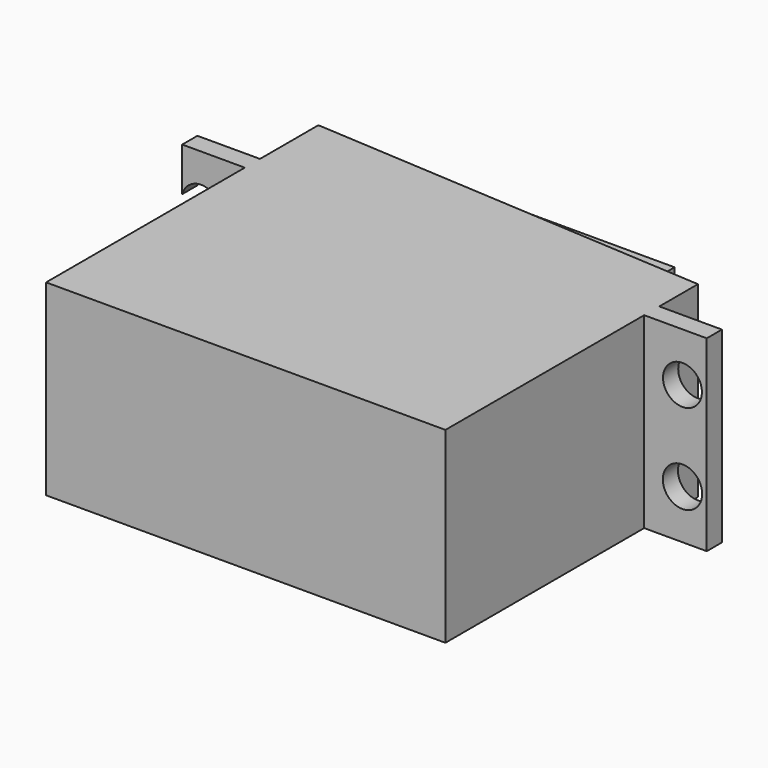
from build123d import *

# Parameters (mm, degrees)
F1_DEPTH = 9.885
F2_DEPTH = 8.905
F3_R     = 2.05
F3_R_2   = 2.075
F4_DEPTH = 25
F5_R     = 0.9
F6_DEPTH = 4.13


# Not quite as in the source:
# - a feature names something its author has since deleted; it is built from what else it names


with BuildPart() as f1:
    # F0 (on Top) → F1 (new body, symmetric)
    with BuildSketch(Plane.XY):
        Polygon((-4.56, 26.2), (-4.56, 0), (37.56, 0), (37.56, 26.2), (44.16, 26.2), (44.16, 28.2), (37.56, 28.2), (37.56, 33.2866495507), (33, 33.56957638), (0, 35.6170731707), (-4.56, 35.9), (-4.56, 28.2), (-11.16, 28.2), (-11.16, 26.2), align=None)
    extrude(amount=F1_DEPTH, both=True)

    # F0 (on Top) → F2 (join, symmetric)
    with BuildSketch(Plane.XY):
        Polygon((0, 35.9067581594), (0, 35.6170731707), (33, 33.56957638), (33, 35.9067581594), align=None)
    extrude(amount=F2_DEPTH, both=True)

    # F3 (on face) → F4 (cut)
    with BuildSketch(Plane(origin=(0, 28.2, 0), x_dir=(-1, 0, 0), z_dir=(0, 1, 0))):
        with Locations((9.16, -4.725)):
            Circle(F3_R)
        with Locations((9.16, 4.725)):
            Circle(F3_R_2)
        with Locations((-41.6, 4.725)):
            Circle(F3_R)
        with Locations((-41.6, -4.725)):
            Circle(F3_R_2)
    extrude(amount=-F4_DEPTH, mode=Mode.SUBTRACT)


with BuildPart() as f6:
    # F5 (on face) → F6 (new body)
    with BuildSketch(Plane(origin=(0, 35.9067581594, 0), x_dir=(-1, 0, 0), z_dir=(0, 1, 0))):
        with BuildLine():
            ThreePointArc((-28.6899656189, 1.033338959), (-28.6260791291, 1.1874039543), (-28.5534413217, 1.3375414089))
            Line((-28.5534413217, 1.3375414089), (-28.8418312249, 1.2937666255))
            Line((-28.8418312249, 1.2937666255), (-28.6899656189, 1.033338959))
        make_face()
        with BuildLine():
            ThreePointArc((-28.5390874953, 1.3648001419), (-28.4563953056, 1.5096431883), (-28.3655130563, 1.6494928329))
            Line((-28.3655130563, 1.6494928329), (-28.6571153541, 1.6422080659))
            Line((-28.6571153541, 1.6422080659), (-28.5390874953, 1.3648001419))
        make_face()
        with BuildLine():
            ThreePointArc((-28.347855989, 1.6747376112), (-28.2476622045, 1.8080744474), (-28.1399687808, 1.9354307696))
            Line((-28.1399687808, 1.9354307696), (-28.4301847307, 1.964750904))
            Line((-28.4301847307, 1.964750904), (-28.347855989, 1.6747376112))
        make_face()
        with BuildLine():
            ThreePointArc((-28.119286935, 1.9582634679), (-28.0031716716, 2.0779912923), (-27.8803654629, 2.1908458069))
            Line((-27.8803654629, 2.1908458069), (-28.1646181862, 2.2563084468))
            Line((-28.1646181862, 2.2563084468), (-28.119286935, 1.9582634679))
        make_face()
        with BuildLine():
            ThreePointArc((-27.8569850038, 2.2109063399), (-27.7267794685, 2.3151369733), (-27.5907972023, 2.4117098971))
            Line((-27.5907972023, 2.4117098971), (-27.8646038636, 2.5122826574))
            Line((-27.8646038636, 2.5122826574), (-27.8569850038, 2.2109063399))
        make_face()
        with BuildLine():
            ThreePointArc((-27.5650868536, 2.4286818982), (-27.4228444656, 2.5157715612), (-27.2758306633, 2.5945398815))
            Line((-27.2758306633, 2.5945398815), (-27.5348731681, 2.7286366698))
            Line((-27.5348731681, 2.7286366698), (-27.5650868536, 2.4286818982))
        make_face()
        with BuildLine():
            ThreePointArc((-27.2481958926, 2.6081556922), (-27.0961598992, 2.6767309287), (-26.9404330564, 2.736452422))
            Line((-26.9404330564, 2.736452422), (-27.1806261495, 2.9019584519))
            Line((-27.1806261495, 2.9019584519), (-27.2481958926, 2.6081556922))
        make_face()
        with BuildLine():
            ThreePointArc((-26.9113096805, 2.7464973129), (-26.7518777802, 2.7954766504), (-26.5898938022, 2.8352094732))
            Line((-26.5898938022, 2.8352094732), (-26.8074494952, 3.0295146156))
            Line((-26.8074494952, 3.0295146156), (-26.9113096805, 2.7464973129))
        make_face()
        with BuildLine():
            ThreePointArc((-26.5597411142, 2.8415250302), (-26.3954276433, 2.8701360355), (-26.2297411142, 2.8892535774))
            Line((-26.2297411142, 2.8892535774), (-26.4212284237, 3.1092935242))
            Line((-26.4212284237, 3.1092935242), (-26.5597411142, 2.8415250302))
        make_face()
        with BuildLine():
            ThreePointArc((-26.1990346399, 2.8917402004), (-26.03243092, 2.8995316607), (-25.8656548153, 2.8977324266))
            Line((-25.8656548153, 2.8977324266), (-26.0280538722, 3.1400370164))
            Line((-26.0280538722, 3.1400370164), (-26.1990346399, 2.8917402004))
        make_face()
        with BuildLine():
            ThreePointArc((-25.8348788143, 2.8963509002), (-25.6686122856, 2.8831999396), (-25.5033767641, 2.8605123045))
            Line((-25.5033767641, 2.8605123045), (-25.6341264382, 3.1212602492))
            Line((-25.6341264382, 3.1212602492), (-25.8348788143, 2.8963509002))
        make_face()
        with BuildLine():
            ThreePointArc((-25.4730165922, 2.8552844161), (-25.3097093771, 2.8213984331), (-25.1486203018, 2.7781801945))
            Line((-25.1486203018, 2.7781801945), (-25.2456585926, 3.0532593432))
            Line((-25.2456585926, 3.0532593432), (-25.4730165922, 2.8552844161))
        make_face()
        with BuildLine():
            ThreePointArc((-25.1191547571, 2.7691883911), (-24.961382308, 2.7151017878), (-24.8069801497, 2.6520345233))
            Line((-24.8069801497, 2.6520345233), (-24.8687767054, 2.9371067135))
            Line((-24.8687767054, 2.9371067135), (-25.1191547571, 2.7691883911))
        make_face()
        with BuildLine():
            ThreePointArc((-24.7788739214, 2.6394206109), (-24.6291244041, 2.5659863655), (-24.4838441771, 2.4840646834))
            Line((-24.4838441771, 2.4840646834), (-24.5094244291, 2.7746341564))
            Line((-24.5094244291, 2.7746341564), (-24.7788739214, 2.6394206109))
        make_face()
        with BuildLine():
            ThreePointArc((-24.4575405173, 2.468027591), (-24.3181755711, 2.3764038053), (-24.1843084314, 2.2769196595))
            Line((-24.1843084314, 2.2769196595), (-24.1732689638, 2.5684039611))
            Line((-24.1732689638, 2.5684039611), (-24.4575405173, 2.468027591))
        make_face()
        with BuildLine():
            ThreePointArc((-24.1602221644, 2.2577123016), (-24.0334396577, 2.1493439375), (-23.9130967701, 2.0338662524))
            Line((-23.9130967701, 2.0338662524), (-23.865611682, 2.3216685011))
            Line((-23.865611682, 2.3216685011), (-24.1602221644, 2.2577123016))
        make_face()
        with BuildLine():
            ThreePointArc((-23.8916077508, 2.0117915406), (-23.7794071196, 1.8883876318), (-23.6744863633, 1.7587375596))
            Line((-23.6744863633, 1.7587375596), (-23.5913045228, 2.0383189419))
            Line((-23.5913045228, 2.0383189419), (-23.8916077508, 2.0117915406))
        make_face()
        with BuildLine():
            ThreePointArc((-23.6559334863, 1.7341436251), (-23.5600842015, 1.5976503252), (-23.4722402395, 1.4558725248))
            Line((-23.4722402395, 1.4558725248), (-23.354673474, 1.7228238754))
            Line((-23.354673474, 1.7228238754), (-23.6559334863, 1.7341436251))
        make_face()
        with BuildLine():
            ThreePointArc((-23.4569160948, 1.4291472288), (-23.3789297569, 1.2817171185), (-23.3095479409, 1.1300475106))
            Line((-23.3095479409, 1.1300475106), (-23.1594503485, 1.3801588472))
            Line((-23.1594503485, 1.3801588472), (-23.4569160948, 1.4291472288))
        make_face()
        with BuildLine():
            ThreePointArc((-23.2976941995, 1.101612327), (-23.2388006996, 0.9455704672), (-23.1889752223, 0.7864009721))
            Line((-23.1889752223, 0.7864009721), (-23.0087139317, 1.0157278895))
            Line((-23.0087139317, 1.0157278895), (-23.2976941995, 1.101612327))
        make_face()
        with BuildLine():
            ThreePointArc((-23.1807788247, 0.7567043406), (-23.1419069485, 0.5945116047), (-23.1124235875, 0.4303524205))
            Line((-23.1124235875, 0.4303524205), (-22.9048414269, 0.6352782962))
            Line((-22.9048414269, 0.6352782962), (-23.1807788247, 0.7567043406))
        make_face()
        with BuildLine():
            ThreePointArc((-23.1080137957, 0.3998626748), (-23.0897765759, 0.2340769392), (-23.0811003014, 0.0675169542))
            Line((-23.0811003014, 0.0675169542), (-22.8494709655, 0.2448099847))
            Line((-22.8494709655, 0.2448099847), (-23.1080137957, 0.3998626748))
        make_face()
        with BuildLine():
            ThreePointArc((-23.0805466606, 0.0367149358), (-23.0803723456, 0.0183578357), (-23.0803142399, 0))
            ThreePointArc((-23.0803142399, 0), (-23.0841130057, -0.1483860211), (-23.0954993511, -0.2963832949))
            Line((-23.0954993511, -0.2963832949), (-22.8434757729, -0.1495191265))
            Line((-22.8434757729, -0.1495191265), (-23.0805466606, 0.0367149358))
        make_face()
        with BuildLine():
            Line((-22.8869503967, -0.5414902318), (-23.0988105925, -0.3270118197))
            ThreePointArc((-23.0988105925, -0.3270118197), (-23.1223755644, -0.4921245038), (-23.1553936549, -0.6556094023))
            Line((-23.1553936549, -0.6556094023), (-22.8869503967, -0.5414902318))
        make_face()
        with BuildLine():
            Line((-22.9792092163, -0.9249217126), (-23.1625175582, -0.6855814035))
            ThreePointArc((-23.1625175582, -0.6855814035), (-23.2065908198, -0.8464386506), (-23.2598386438, -1.0044961578))
            Line((-23.2598386438, -1.0044961578), (-22.9792092163, -0.9249217126))
        make_face()
        with BuildLine():
            Line((-23.1187972548, -1.2937666255), (-23.2706628609, -1.033338959))
            ThreePointArc((-23.2706628609, -1.033338959), (-23.3345493506, -1.1874039543), (-23.407187158, -1.3375414089))
            Line((-23.407187158, -1.3375414089), (-23.1187972548, -1.2937666255))
        make_face()
        with BuildLine():
            Line((-23.3035131256, -1.6422080659), (-23.4215409844, -1.3648001419))
            ThreePointArc((-23.4215409844, -1.3648001419), (-23.5042331741, -1.5096431883), (-23.5951154234, -1.6494928329))
            Line((-23.5951154234, -1.6494928329), (-23.3035131256, -1.6422080659))
        make_face()
        with BuildLine():
            Line((-23.530443749, -1.964750904), (-23.6127724907, -1.6747376112))
            ThreePointArc((-23.6127724907, -1.6747376112), (-23.7129662752, -1.8080744474), (-23.820659699, -1.9354307696))
            Line((-23.820659699, -1.9354307696), (-23.530443749, -1.964750904))
        make_face()
        with BuildLine():
            Line((-23.7960102935, -2.2563084468), (-23.8413415448, -1.9582634679))
            ThreePointArc((-23.8413415448, -1.9582634679), (-23.9574568082, -2.0779912923), (-24.0802630168, -2.1908458069))
            Line((-24.0802630168, -2.1908458069), (-23.7960102935, -2.2563084468))
        make_face()
        with BuildLine():
            Line((-24.0960246161, -2.5122826574), (-24.1036434759, -2.2109063399))
            ThreePointArc((-24.1036434759, -2.2109063399), (-24.2338490112, -2.3151369733), (-24.3698312774, -2.4117098971))
            Line((-24.3698312774, -2.4117098971), (-24.0960246161, -2.5122826574))
        make_face()
        with BuildLine():
            Line((-24.4257553117, -2.7286366698), (-24.3955416261, -2.4286818982))
            ThreePointArc((-24.3955416261, -2.4286818982), (-24.5377840142, -2.5157715612), (-24.6847978164, -2.5945398815))
            Line((-24.6847978164, -2.5945398815), (-24.4257553117, -2.7286366698))
        make_face()
        with BuildLine():
            Line((-24.7800023302, -2.9019584519), (-24.7124325872, -2.6081556922))
            ThreePointArc((-24.7124325872, -2.6081556922), (-24.8644685805, -2.6767309287), (-25.0201954233, -2.736452422))
            Line((-25.0201954233, -2.736452422), (-24.7800023302, -2.9019584519))
        make_face()
        with BuildLine():
            Line((-25.1531789846, -3.0295146156), (-25.0493187992, -2.7464973129))
            ThreePointArc((-25.0493187992, -2.7464973129), (-25.2087506995, -2.7954766504), (-25.3707346775, -2.8352094732))
            Line((-25.3707346775, -2.8352094732), (-25.1531789846, -3.0295146156))
        make_face()
        with BuildLine():
            Line((-25.539400056, -3.1092935242), (-25.4008873656, -2.8415250302))
            ThreePointArc((-25.4008873656, -2.8415250302), (-25.5652008364, -2.8701360355), (-25.7308873656, -2.8892535774))
            Line((-25.7308873656, -2.8892535774), (-25.539400056, -3.1092935242))
        make_face()
        with BuildLine():
            Line((-25.9325746075, -3.1400370164), (-25.7615938398, -2.8917402004))
            ThreePointArc((-25.7615938398, -2.8917402004), (-25.9281975597, -2.8995316607), (-26.0949736644, -2.8977324266))
            Line((-26.0949736644, -2.8977324266), (-25.9325746075, -3.1400370164))
        make_face()
        with BuildLine():
            Line((-26.7149698872, -3.0532593432), (-26.4876118875, -2.8552844161))
            ThreePointArc((-26.4876118875, -2.8552844161), (-26.6509191026, -2.8213984331), (-26.8120081779, -2.7781801945))
            Line((-26.8120081779, -2.7781801945), (-26.7149698872, -3.0532593432))
        make_face()
        with BuildLine():
            ThreePointArc((-28.7981109215, 0.6855814035), (-28.7540376599, 0.8464386506), (-28.7007898359, 1.0044961578))
            Line((-28.7007898359, 1.0044961578), (-28.9814192634, 0.9249217126))
            Line((-28.9814192634, 0.9249217126), (-28.7981109215, 0.6855814035))
        make_face()
        with BuildLine():
            ThreePointArc((-28.8618178872, 0.3270118197), (-28.8382529153, 0.4921245038), (-28.8052348249, 0.6556094023))
            Line((-28.8052348249, 0.6556094023), (-29.073678083, 0.5414902318))
            Line((-29.073678083, 0.5414902318), (-28.8618178872, 0.3270118197))
        make_face()
        with BuildLine():
            Line((-29.1111575142, -0.2448099847), (-28.852614684, -0.3998626748))
            ThreePointArc((-28.852614684, -0.3998626748), (-28.8708519038, -0.2340769392), (-28.8795281783, -0.0675169542))
            Line((-28.8795281783, -0.0675169542), (-29.1111575142, -0.2448099847))
        make_face()
        with BuildLine():
            Line((-29.0557870528, -0.6352782962), (-28.779849655, -0.7567043406))
            ThreePointArc((-28.779849655, -0.7567043406), (-28.8187215313, -0.5945116047), (-28.8482048923, -0.4303524205))
            Line((-28.8482048923, -0.4303524205), (-29.0557870528, -0.6352782962))
        make_face()
        with BuildLine():
            Line((-28.951914548, -1.0157278895), (-28.6629342803, -1.101612327))
            ThreePointArc((-28.6629342803, -1.101612327), (-28.7218277802, -0.9455704672), (-28.7716532574, -0.7864009721))
            Line((-28.7716532574, -0.7864009721), (-28.951914548, -1.0157278895))
        make_face()
        with BuildLine():
            Line((-28.8011781312, -1.3801588472), (-28.5037123849, -1.4291472288))
            ThreePointArc((-28.5037123849, -1.4291472288), (-28.5816987228, -1.2817171185), (-28.6510805388, -1.1300475106))
            Line((-28.6510805388, -1.1300475106), (-28.8011781312, -1.3801588472))
        make_face()
        with BuildLine():
            ThreePointArc((-23.0954993511, -0.2963832949), (-23.0841130057, -0.1483860211), (-23.0803142399, 0))
            ThreePointArc((-23.0803142399, 0), (-23.0803723456, 0.0183578357), (-23.0805466606, 0.0367149358))
            ThreePointArc((-23.0805466606, 0.0367149358), (-23.0807825791, 0.0521166802), (-23.0811003014, 0.0675169542))
            ThreePointArc((-23.0811003014, 0.0675169542), (-23.0897765759, 0.2340769392), (-23.1080137957, 0.3998626748))
            ThreePointArc((-23.1080137957, 0.3998626748), (-23.1101782044, 0.4151134034), (-23.1124235875, 0.4303524205))
            ThreePointArc((-23.1124235875, 0.4303524205), (-23.1419069485, 0.5945116047), (-23.1807788247, 0.7567043406))
            ThreePointArc((-23.1807788247, 0.7567043406), (-23.1848375894, 0.7715635404), (-23.1889752223, 0.7864009721))
            ThreePointArc((-23.1889752223, 0.7864009721), (-23.2388006996, 0.9455704672), (-23.2976941995, 1.101612327))
            ThreePointArc((-23.2976941995, 1.101612327), (-23.3035833112, 1.1158456593), (-23.3095479409, 1.1300475106))
            ThreePointArc((-23.3095479409, 1.1300475106), (-23.3789297569, 1.2817171185), (-23.4569160948, 1.4291472288))
            ThreePointArc((-23.4569160948, 1.4291472288), (-23.4645426787, 1.4425302257), (-23.4722402395, 1.4558725248))
            ThreePointArc((-23.4722402395, 1.4558725248), (-23.5600842015, 1.5976503252), (-23.6559334863, 1.7341436251))
            ThreePointArc((-23.6559334863, 1.7341436251), (-23.6651772666, 1.7464652287), (-23.6744863633, 1.7587375596))
            ThreePointArc((-23.6744863633, 1.7587375596), (-23.7794071196, 1.8883876318), (-23.8916077508, 2.0117915406))
            ThreePointArc((-23.8916077508, 2.0117915406), (-23.9023229475, 2.0228574317), (-23.9130967701, 2.0338662524))
            ThreePointArc((-23.9130967701, 2.0338662524), (-24.0334396577, 2.1493439375), (-24.1602221644, 2.2577123016))
            ThreePointArc((-24.1602221644, 2.2577123016), (-24.1722397925, 2.2673479646), (-24.1843084314, 2.2769196595))
            ThreePointArc((-24.1843084314, 2.2769196595), (-24.3181755711, 2.3764038053), (-24.4575405173, 2.468027591))
            ThreePointArc((-24.4575405173, 2.468027591), (-24.4706710516, 2.4760810657), (-24.4838441771, 2.4840646834))
            ThreePointArc((-24.4838441771, 2.4840646834), (-24.6291244041, 2.5659863655), (-24.7788739214, 2.6394206109))
            ThreePointArc((-24.7788739214, 2.6394206109), (-24.7929102856, 2.6457648893), (-24.8069801497, 2.6520345233))
            ThreePointArc((-24.8069801497, 2.6520345233), (-24.961382308, 2.7151017878), (-25.1191547571, 2.7691883911))
            ThreePointArc((-25.1191547571, 2.7691883911), (-25.1338755892, 2.77372342), (-25.1486203018, 2.7781801945))
            ThreePointArc((-25.1486203018, 2.7781801945), (-25.3097093771, 2.8213984331), (-25.4730165922, 2.8552844161))
            ThreePointArc((-25.4730165922, 2.8552844161), (-25.4881897361, 2.8579386755), (-25.5033767641, 2.8605123045))
            ThreePointArc((-25.5033767641, 2.8605123045), (-25.6686122856, 2.8831999396), (-25.8348788143, 2.8963509002))
            ThreePointArc((-25.8348788143, 2.8963509002), (-25.8502649803, 2.8970825308), (-25.8656548153, 2.8977324266))
            ThreePointArc((-25.8656548153, 2.8977324266), (-26.03243092, 2.8995316607), (-26.1990346399, 2.8917402004))
            ThreePointArc((-26.1990346399, 2.8917402004), (-26.214391179, 2.8905376639), (-26.2297411142, 2.8892535774))
            ThreePointArc((-26.2297411142, 2.8892535774), (-26.3954276433, 2.8701360355), (-26.5597411142, 2.8415250302))
            ThreePointArc((-26.5597411142, 2.8415250302), (-26.5748258446, 2.8384072914), (-26.5898938022, 2.8352094732))
            ThreePointArc((-26.5898938022, 2.8352094732), (-26.7518777802, 2.7954766504), (-26.9113096805, 2.7464973129))
            ThreePointArc((-26.9113096805, 2.7464973129), (-26.925884707, 2.7415135403), (-26.9404330564, 2.736452422))
            ThreePointArc((-26.9404330564, 2.736452422), (-27.0961598992, 2.6767309287), (-27.2481958926, 2.6081556922))
            ThreePointArc((-27.2481958926, 2.6081556922), (-27.2620313583, 2.601384483), (-27.2758306633, 2.5945398815))
            ThreePointArc((-27.2758306633, 2.5945398815), (-27.4228444656, 2.5157715612), (-27.5650868536, 2.4286818982))
            ThreePointArc((-27.5650868536, 2.4286818982), (-27.577964565, 2.4202300384), (-27.5907972023, 2.4117098971))
            ThreePointArc((-27.5907972023, 2.4117098971), (-27.7267794685, 2.3151369733), (-27.8569850038, 2.2109063399))
            ThreePointArc((-27.8569850038, 2.2109063399), (-27.8687018717, 2.2009071203), (-27.8803654629, 2.1908458069))
            ThreePointArc((-27.8803654629, 2.1908458069), (-28.0031716716, 2.0779912923), (-28.119286935, 1.9582634679))
            ThreePointArc((-28.119286935, 1.9582634679), (-28.1296581773, 1.9468745821), (-28.1399687808, 1.9354307696))
            ThreePointArc((-28.1399687808, 1.9354307696), (-28.2476622045, 1.8080744474), (-28.347855989, 1.6747376112))
            ThreePointArc((-28.347855989, 1.6747376112), (-28.3567180451, 1.6621386688), (-28.3655130563, 1.6494928329))
            ThreePointArc((-28.3655130563, 1.6494928329), (-28.4563953056, 1.5096431883), (-28.5390874953, 1.3648001419))
            ThreePointArc((-28.5390874953, 1.3648001419), (-28.5463006053, 1.3511898358), (-28.5534413217, 1.3375414089))
            ThreePointArc((-28.5534413217, 1.3375414089), (-28.6260791291, 1.1874039543), (-28.6899656189, 1.033338959))
            ThreePointArc((-28.6899656189, 1.033338959), (-28.6954160277, 1.0189319319), (-28.7007898359, 1.0044961578))
            ThreePointArc((-28.7007898359, 1.0044961578), (-28.7540376599, 0.8464386506), (-28.7981109215, 0.6855814035))
            ThreePointArc((-28.7981109215, 0.6855814035), (-28.8017126729, 0.6706048627), (-28.8052348249, 0.6556094023))
            ThreePointArc((-28.8052348249, 0.6556094023), (-28.8382529153, 0.4921245038), (-28.8618178872, 0.3270118197))
            ThreePointArc((-28.8618178872, 0.3270118197), (-28.8635141795, 0.3117019543), (-28.8651291286, 0.2963832949))
            ThreePointArc((-28.8651291286, 0.2963832949), (-28.8773967706, 0.1300492596), (-28.8800818191, -0.0367149358))
            ThreePointArc((-28.8800818191, -0.0367149358), (-28.8798459006, -0.0521166802), (-28.8795281783, -0.0675169542))
            ThreePointArc((-28.8795281783, -0.0675169542), (-28.8708519038, -0.2340769392), (-28.852614684, -0.3998626748))
            ThreePointArc((-28.852614684, -0.3998626748), (-28.8504502754, -0.4151134034), (-28.8482048923, -0.4303524205))
            ThreePointArc((-28.8482048923, -0.4303524205), (-28.8187215313, -0.5945116047), (-28.779849655, -0.7567043406))
            ThreePointArc((-28.779849655, -0.7567043406), (-28.7757908903, -0.7715635403), (-28.7716532574, -0.7864009721))
            ThreePointArc((-28.7716532574, -0.7864009721), (-28.7218277802, -0.9455704672), (-28.6629342803, -1.101612327))
            ThreePointArc((-28.6629342803, -1.101612327), (-28.6570451685, -1.1158456593), (-28.6510805388, -1.1300475106))
            ThreePointArc((-28.6510805388, -1.1300475106), (-28.5816987228, -1.2817171185), (-28.5037123849, -1.4291472288))
            ThreePointArc((-28.5037123849, -1.4291472288), (-28.496085801, -1.4425302257), (-28.4883882403, -1.4558725248))
            ThreePointArc((-28.4883882403, -1.4558725248), (-28.4005442782, -1.5976503252), (-28.3046949934, -1.7341436251))
            ThreePointArc((-28.3046949934, -1.7341436251), (-28.2954512131, -1.7464652287), (-28.2861421165, -1.7587375596))
            ThreePointArc((-28.2861421165, -1.7587375596), (-28.1812213601, -1.8883876318), (-28.0690207289, -2.0117915406))
            ThreePointArc((-28.0690207289, -2.0117915406), (-28.0583055322, -2.0228574317), (-28.0475317096, -2.0338662524))
            ThreePointArc((-28.0475317096, -2.0338662524), (-27.927188822, -2.1493439375), (-27.8004063153, -2.2577123016))
            ThreePointArc((-27.8004063153, -2.2577123016), (-27.7883886872, -2.2673479646), (-27.7763200483, -2.2769196595))
            ThreePointArc((-27.7763200483, -2.2769196595), (-27.6424529087, -2.3764038053), (-27.5030879625, -2.468027591))
            ThreePointArc((-27.5030879625, -2.468027591), (-27.4899574281, -2.4760810657), (-27.4767843026, -2.4840646834))
            ThreePointArc((-27.4767843026, -2.4840646834), (-27.3315040756, -2.5659863655), (-27.1817545583, -2.6394206109))
            ThreePointArc((-27.1817545583, -2.6394206109), (-27.1677181942, -2.6457648893), (-27.15364833, -2.6520345233))
            ThreePointArc((-27.15364833, -2.6520345233), (-26.9992461717, -2.7151017878), (-26.8414737227, -2.7691883911))
            ThreePointArc((-26.8414737227, -2.7691883911), (-26.8267528905, -2.77372342), (-26.8120081779, -2.7781801945))
            ThreePointArc((-26.8120081779, -2.7781801945), (-26.6509191026, -2.8213984331), (-26.4876118875, -2.8552844161))
            ThreePointArc((-26.4876118875, -2.8552844161), (-26.4724387437, -2.8579386755), (-26.4572517156, -2.8605123045))
            ThreePointArc((-26.4572517156, -2.8605123045), (-26.2920161942, -2.8831999396), (-26.1257496654, -2.8963509002))
            ThreePointArc((-26.1257496654, -2.8963509002), (-26.1103634994, -2.8970825308), (-26.0949736644, -2.8977324266))
            ThreePointArc((-26.0949736644, -2.8977324266), (-25.9281975597, -2.8995316607), (-25.7615938398, -2.8917402004))
            ThreePointArc((-25.7615938398, -2.8917402004), (-25.7462373007, -2.8905376639), (-25.7308873656, -2.8892535774))
            ThreePointArc((-25.7308873656, -2.8892535774), (-25.5652008364, -2.8701360355), (-25.4008873656, -2.8415250302))
            ThreePointArc((-25.4008873656, -2.8415250302), (-25.3858026351, -2.8384072914), (-25.3707346775, -2.8352094732))
            ThreePointArc((-25.3707346775, -2.8352094732), (-25.2087506995, -2.7954766504), (-25.0493187992, -2.7464973129))
            ThreePointArc((-25.0493187992, -2.7464973129), (-25.0347437727, -2.7415135403), (-25.0201954233, -2.736452422))
            ThreePointArc((-25.0201954233, -2.736452422), (-24.8644685805, -2.6767309287), (-24.7124325872, -2.6081556922))
            ThreePointArc((-24.7124325872, -2.6081556922), (-24.6985971214, -2.601384483), (-24.6847978164, -2.5945398815))
            ThreePointArc((-24.6847978164, -2.5945398815), (-24.5377840142, -2.5157715612), (-24.3955416261, -2.4286818982))
            ThreePointArc((-24.3955416261, -2.4286818982), (-24.3826639147, -2.4202300384), (-24.3698312774, -2.4117098971))
            ThreePointArc((-24.3698312774, -2.4117098971), (-24.2338490112, -2.3151369733), (-24.1036434759, -2.2109063399))
            ThreePointArc((-24.1036434759, -2.2109063399), (-24.091926608, -2.2009071203), (-24.0802630168, -2.1908458069))
            ThreePointArc((-24.0802630168, -2.1908458069), (-23.9574568082, -2.0779912923), (-23.8413415448, -1.9582634679))
            ThreePointArc((-23.8413415448, -1.9582634679), (-23.8309703024, -1.9468745821), (-23.820659699, -1.9354307696))
            ThreePointArc((-23.820659699, -1.9354307696), (-23.7129662752, -1.8080744474), (-23.6127724907, -1.6747376112))
            ThreePointArc((-23.6127724907, -1.6747376112), (-23.6039104346, -1.6621386688), (-23.5951154234, -1.6494928329))
            ThreePointArc((-23.5951154234, -1.6494928329), (-23.5042331741, -1.5096431883), (-23.4215409844, -1.3648001419))
            ThreePointArc((-23.4215409844, -1.3648001419), (-23.4143278744, -1.3511898358), (-23.407187158, -1.3375414089))
            ThreePointArc((-23.407187158, -1.3375414089), (-23.3345493506, -1.1874039543), (-23.2706628609, -1.033338959))
            ThreePointArc((-23.2706628609, -1.033338959), (-23.265212452, -1.0189319319), (-23.2598386438, -1.0044961578))
            ThreePointArc((-23.2598386438, -1.0044961578), (-23.2065908198, -0.8464386506), (-23.1625175582, -0.6855814035))
            ThreePointArc((-23.1625175582, -0.6855814035), (-23.1589158068, -0.6706048627), (-23.1553936549, -0.6556094023))
            ThreePointArc((-23.1553936549, -0.6556094023), (-23.1223755644, -0.4921245038), (-23.0988105925, -0.3270118197))
            ThreePointArc((-23.0988105925, -0.3270118197), (-23.0971143003, -0.3117019543), (-23.0954993511, -0.2963832949))
        make_face()
        with Locations((-25.9803142399, 0)):
            Circle(F5_R, mode=Mode.SUBTRACT)
        with BuildLine():
            Line((-28.6059550057, -1.7228238754), (-28.3046949934, -1.7341436251))
            ThreePointArc((-28.3046949934, -1.7341436251), (-28.4005442782, -1.5976503252), (-28.4883882403, -1.4558725248))
            Line((-28.4883882403, -1.4558725248), (-28.6059550057, -1.7228238754))
        make_face()
        with BuildLine():
            Line((-28.3693239569, -2.0383189419), (-28.0690207289, -2.0117915406))
            ThreePointArc((-28.0690207289, -2.0117915406), (-28.1812213601, -1.8883876318), (-28.2861421165, -1.7587375596))
            Line((-28.2861421165, -1.7587375596), (-28.3693239569, -2.0383189419))
        make_face()
        with BuildLine():
            Line((-28.0950167977, -2.3216685011), (-27.8004063153, -2.2577123016))
            ThreePointArc((-27.8004063153, -2.2577123016), (-27.927188822, -2.1493439375), (-28.0475317096, -2.0338662524))
            Line((-28.0475317096, -2.0338662524), (-28.0950167977, -2.3216685011))
        make_face()
        with BuildLine():
            Line((-27.7873595159, -2.5684039611), (-27.5030879625, -2.468027591))
            ThreePointArc((-27.5030879625, -2.468027591), (-27.6424529087, -2.3764038053), (-27.7763200483, -2.2769196595))
            Line((-27.7763200483, -2.2769196595), (-27.7873595159, -2.5684039611))
        make_face()
        with BuildLine():
            Line((-27.4512040506, -2.7746341564), (-27.1817545583, -2.6394206109))
            ThreePointArc((-27.1817545583, -2.6394206109), (-27.3315040756, -2.5659863655), (-27.4767843026, -2.4840646834))
            Line((-27.4767843026, -2.4840646834), (-27.4512040506, -2.7746341564))
        make_face()
        with BuildLine():
            Line((-27.0918517744, -2.9371067135), (-26.8414737227, -2.7691883911))
            ThreePointArc((-26.8414737227, -2.7691883911), (-26.9992461717, -2.7151017878), (-27.15364833, -2.6520345233))
            Line((-27.15364833, -2.6520345233), (-27.0918517744, -2.9371067135))
        make_face()
        with BuildLine():
            Line((-26.3265020416, -3.1212602492), (-26.1257496654, -2.8963509002))
            ThreePointArc((-26.1257496654, -2.8963509002), (-26.2920161942, -2.8831999396), (-26.4572517156, -2.8605123045))
            Line((-26.4572517156, -2.8605123045), (-26.3265020416, -3.1212602492))
        make_face()
        with BuildLine():
            ThreePointArc((-28.8800818191, -0.0367149358), (-28.8773967706, 0.1300492596), (-28.8651291286, 0.2963832949))
            Line((-28.8651291286, 0.2963832949), (-29.1171527068, 0.1495191265))
            Line((-29.1171527068, 0.1495191265), (-28.8800818191, -0.0367149358))
        make_face()
    extrude(amount=F6_DEPTH)


solid = Compound([f1.part, f6.part])
